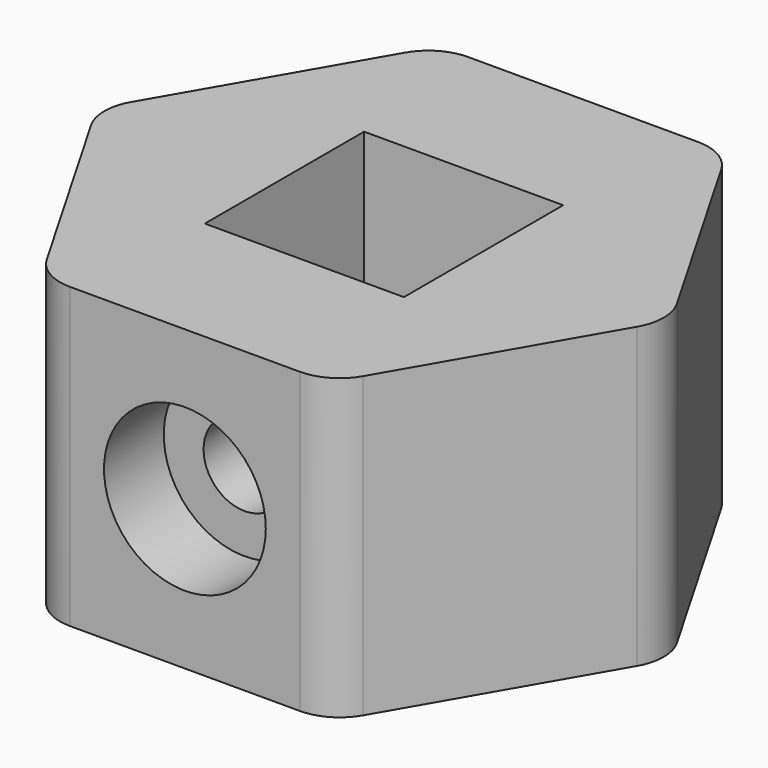
from build123d import *

# Parameters (mm, degrees)
F0_W           = 8
F0_H           = 8
F1_DEPTH       = 12
F3_D           = 3.3
F3_DEPTH       = 12
F3_CBORE_D     = 6.5
F3_CBORE_DEPTH = 3
F3_TIP         = 0.9914200214
F4_R           = 2


with BuildPart() as f1:
    # F0 (on Top) → F1 (new body)
    with BuildSketch(Plane.XY):
        Polygon((5.7735026919, -10), (11.5470053838, 0), (5.7735026919, 10), (-5.7735026919, 10), (-11.5470053838, 0), (-5.7735026919, -10), align=None)
        Rectangle(F0_W, F0_H, mode=Mode.SUBTRACT)
    extrude(amount=F1_DEPTH)

    # F3
    with Locations(Plane.XZ.offset(10)):
        with Locations((0, 6)):
            CounterBoreHole(F3_D / 2, F3_CBORE_D / 2, F3_CBORE_DEPTH, depth=F3_DEPTH)
            with Locations((0, 0, -(F3_DEPTH + F3_TIP / 2))):  # 118° drill point
                Cone(0, F3_D / 2, F3_TIP, mode=Mode.SUBTRACT)

    # F4
    f4_edges = [f1.edges().sort_by_distance(p)[0] for p in [
        (-11.547005, 0, 6),
        (-5.773503, -10, 6),
        (5.773503, -10, 6),
        (11.547005, 0, 6),
        (5.773503, 10, 6),
        (-5.773503, 10, 6),
    ]]
    fillet(f4_edges, radius=F4_R)


solid = f1.part
